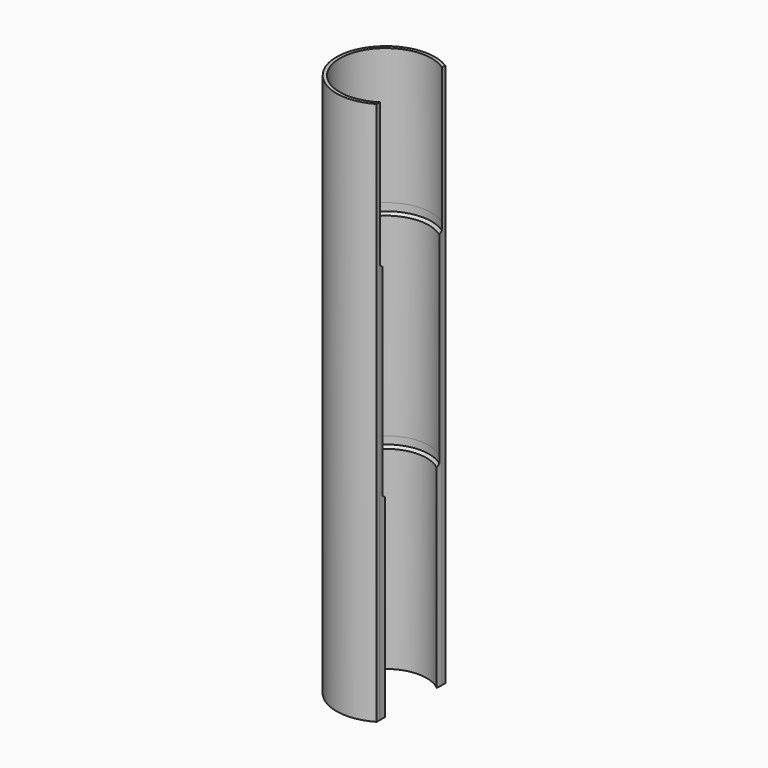
from build123d import *

# Parameters (mm, degrees)
F1_DEPTH     = 80
F2_DEPTH     = 60
F3_DEPTH     = 30
F4_T4_ANGLE  = 321.2915133738
F4_S5_R      = 6.75
F4_T6_DEPTH  = 13
F4_T10_ANGLE = 330.397154177
F4_S11_R     = 6.3724602388
F4_T12_DEPTH = 12


# Not quite as in the source:
# - a fillet or chamfer that OpenCascade refuses, or shapes differently, is made with other operations: its cross-section is extruded or revolved along the edge and cut away or added


with BuildPart() as f1:
    # F0 (on Top) → F1 (new body)
    with BuildSketch(Plane.XY):
        with BuildLine():
            ThreePointArc((3.6719317522, -5.6638694553), (-6.7494746232, 0.0842158591), (3.8121072666, 5.5704881463))
            Line((3.8121072666, 5.5704881463), (3.8276649179, 6.1572300003))
            ThreePointArc((3.8276649179, 6.1572300003), (-7.2494177613, 0.091881022), (3.6703837587, -6.2522622357))
            Line((3.6703837587, -6.2522622357), (3.6719317522, -5.6638694553))
        make_face()
    extrude(amount=F1_DEPTH)

    # F0 (on Top) → F2 (join)
    with BuildSketch(Plane.XY):
        with BuildLine():
            Line((3.7829003883, 5.1256385395), (3.8121072666, 5.5704881463))
            ThreePointArc((3.8121072666, 5.5704881463), (-6.7494746232, 0.0842158591), (3.6719317522, -5.6638694553))
            Line((3.6719317522, -5.6638694553), (3.6728513037, -5.2038225677))
            ThreePointArc((3.6728513037, -5.2038225677), (-6.3764069894, 0.0685580429), (3.7829003883, 5.1256385395))
        make_face()
    extrude(amount=F2_DEPTH)

    # F0 (on Top) → F3 (join)
    with BuildSketch(Plane.XY):
        with BuildLine():
            Line((3.75369351, 4.6807889327), (3.7829003883, 5.1256385395))
            ThreePointArc((3.7829003883, 5.1256385395), (-6.3764069894, 0.0685580429), (3.6728513037, -5.2038225677))
            Line((3.6728513037, -5.2038225677), (3.6737708552, -4.7437756801))
            ThreePointArc((3.6737708552, -4.7437756801), (-5.9997842678, 0.0508796647), (3.75369351, 4.6807889327))
        make_face()
    extrude(amount=F3_DEPTH)

    # F4: chamfer of 1.5 on 2 edges, made by hand


with BuildPart() as f4_tool2:
    # F4_s3 → F4_t4 (revolve)
    with BuildSketch(Plane(origin=(-0.0002871576, -0.0007904765, 0), x_dir=(0, 0, 1), z_dir=(0.341440213, 0.9399034955, 0))):
        Polygon((60, 7.8681819087), (58.5, 6.3681819087), (60, 6.3681819087), align=None)
    revolve(axis=Axis((-0.004308375, 0.0006703174, 60), (0, 0, -1)), revolution_arc=F4_T4_ANGLE)

    # F4_s5 → F4_t6 (intersect, symmetric)
    with BuildSketch(Plane.XY.offset(59.2)):
        Circle(F4_S5_R)
    extrude(amount=F4_T6_DEPTH, both=True, mode=Mode.INTERSECT)


with BuildPart() as f1_1:
    add(f1.part)

    # F4_t1: cut F4_tool2
    add(f4_tool2.part, mode=Mode.SUBTRACT)


with BuildPart() as f4_tool8:
    # F4_s9 → F4_t10 (revolve)
    with BuildSketch(Plane(origin=(0, 0, 0), x_dir=(0, 0, 1), z_dir=(0.2636591374, 0.9646159128, 0))):
        Polygon((30, 7.5), (28.5, 6), (30, 6), align=None)
    revolve(axis=Axis((0, 0, 30), (0, 0, -1)), revolution_arc=F4_T10_ANGLE)

    # F4_s11 → F4_t12 (intersect, symmetric)
    with BuildSketch(Plane.XY.offset(29.2)):
        with Locations((-0.004308375, 0.0006703174)):
            Circle(F4_S11_R)
    extrude(amount=F4_T12_DEPTH, both=True, mode=Mode.INTERSECT)


with BuildPart() as f1_2:
    add(f1_1.part)

    # F4_t7: cut F4_tool8
    add(f4_tool8.part, mode=Mode.SUBTRACT)


solid = f1_2.part
